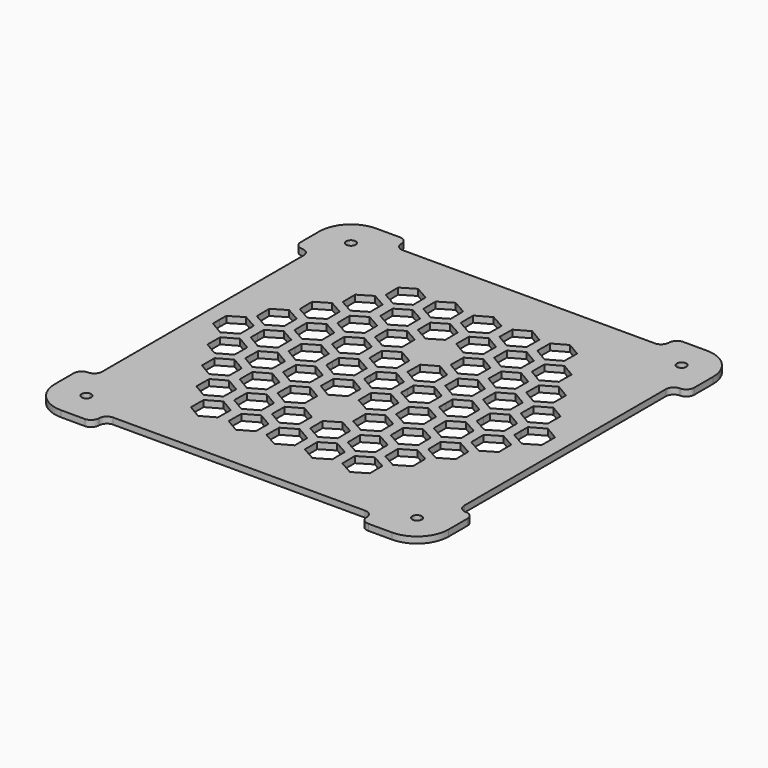
from build123d import *

# Parameters (mm, degrees)
F2_DEPTH = 2
F3_DEPTH = 2
F4_DEPTH = 2
F5_R     = 2.49999
F6_R     = 10


# Not quite as in the source:
# - a fillet or chamfer is up to 0.001 mm smaller than in the source, because OpenCascade refuses the exact size


with BuildPart() as f2:
    # F0 (on Top) → F2 (new body)
    with BuildSketch(Plane.XY):
        Polygon((-57.5, -57.5), (-57.5, -42.5), (-62.5, -42.5), (-62.5, -62.5), (-42.5, -62.5), (-42.5, -57.5), align=None)
        with BuildLine():
            Line((-52.5, -51), (-52.5, -42.5))
            Line((-52.5, -42.5), (-57.5, -42.5))
            Line((-57.5, -42.5), (-57.5, -57.5))
            Line((-57.5, -57.5), (-42.5, -57.5))
            Line((-42.5, -57.5), (-42.5, -52.5))
            Line((-42.5, -52.5), (-51, -52.5))
            ThreePointArc((-51, -52.5), (-53.5606601718, -53.5606601718), (-52.5, -51))
        make_face()
        with BuildLine():
            Line((-42.5, -42.5), (-52.5, -42.5))
            Line((-52.5, -42.5), (-52.5, -51))
            ThreePointArc((-52.5, -51), (-51.4393398282, -51.4393398282), (-51, -52.5))
            Line((-51, -52.5), (-42.5, -52.5))
            Line((-42.5, -52.5), (-42.5, -42.5))
        make_face()
        with BuildLine():
            ThreePointArc((1.078e-07, -52.5), (-37.1231059749, -37.1231060497), (-52.5, 2.1e-09))
            Line((-52.5, 2.1e-09), (-52.5, -42.5))
            Line((-52.5, -42.5), (-42.5, -42.5))
            Line((-42.5, -42.5), (-42.5, -52.5))
            Line((-42.5, -52.5), (1.078e-07, -52.5))
        make_face()
        Polygon((42.5, -52.5), (1.078e-07, -52.5), (-42.5, -52.5), (-42.5, -57.5), (42.5, -57.5), align=None)
        with BuildLine():
            Line((57.5, -42.5), (52.5, -42.5))
            Line((52.5, -42.5), (52.5, -51))
            ThreePointArc((52.5, -51), (53.5606601718, -51.4393398282), (54, -52.5))
            ThreePointArc((54, -52.5), (52.5, -54), (51, -52.5))
            Line((51, -52.5), (42.5, -52.5))
            Line((42.5, -52.5), (42.5, -57.5))
            Line((42.5, -57.5), (57.5, -57.5))
            Line((57.5, -57.5), (57.5, -42.5))
        make_face()
        Polygon((62.5, -42.5), (57.5, -42.5), (57.5, -57.5), (42.5, -57.5), (42.5, -62.5), (62.5, -62.5), align=None)
        with BuildLine():
            Line((52.5, -51), (52.5, -42.5))
            Line((52.5, -42.5), (42.5, -42.5))
            Line((42.5, -42.5), (42.5, -52.5))
            Line((42.5, -52.5), (51, -52.5))
            ThreePointArc((51, -52.5), (51.4393398282, -51.4393398282), (52.5, -51))
        make_face()
        Polygon((52.5, 42.5), (52.5, 0), (52.5, -42.5), (57.5, -42.5), (57.5, 42.5), align=None)
        Polygon((42.5, 62.5), (42.5, 57.5), (57.5, 57.5), (57.5, 42.5), (62.5, 42.5), (62.5, 62.5), align=None)
        with BuildLine():
            Line((42.5, 57.5), (42.5, 52.5))
            Line((42.5, 52.5), (51, 52.5))
            ThreePointArc((51, 52.5), (52.5, 54), (54, 52.5))
            ThreePointArc((54, 52.5), (53.5606601718, 51.4393398282), (52.5, 51))
            Line((52.5, 51), (52.5, 42.5))
            Line((52.5, 42.5), (57.5, 42.5))
            Line((57.5, 42.5), (57.5, 57.5))
            Line((57.5, 57.5), (42.5, 57.5))
        make_face()
        with BuildLine():
            Line((51, 52.5), (42.5, 52.5))
            Line((42.5, 52.5), (42.5, 42.5))
            Line((42.5, 42.5), (52.5, 42.5))
            Line((52.5, 42.5), (52.5, 51))
            ThreePointArc((52.5, 51), (51.4393398282, 51.4393398282), (51, 52.5))
        make_face()
        with BuildLine():
            Line((42.5, 52.5), (0, 52.5))
            ThreePointArc((0, 52.5), (37.1231060123, 37.1231060123), (52.5, 0))
            Line((52.5, 0), (52.5, 42.5))
            Line((52.5, 42.5), (42.5, 42.5))
            Line((42.5, 42.5), (42.5, 52.5))
        make_face()
        with BuildLine():
            ThreePointArc((-52.5, 51), (-53.5606601718, 53.5606601718), (-51, 52.5))
            Line((-51, 52.5), (-42.5, 52.5))
            Line((-42.5, 52.5), (-42.5, 57.5))
            Line((-42.5, 57.5), (-57.5, 57.5))
            Line((-57.5, 57.5), (-57.5, 42.5))
            Line((-57.5, 42.5), (-52.5, 42.5))
            Line((-52.5, 42.5), (-52.5, 51))
        make_face()
        Polygon((-52.5, 2.1e-09), (-52.5, 42.5), (-57.5, 42.5), (-57.5, -42.5), (-52.5, -42.5), align=None)
        with BuildLine():
            Line((0, 52.5), (-42.5, 52.5))
            Line((-42.5, 52.5), (-42.5, 42.5))
            Line((-42.5, 42.5), (-52.5, 42.5))
            Line((-52.5, 42.5), (-52.5, 2.1e-09))
            ThreePointArc((-52.5, 2.1e-09), (-37.1231060115, 37.123106013), (0, 52.5))
        make_face()
        Polygon((-42.5, 57.5), (-42.5, 52.5), (0, 52.5), (42.5, 52.5), (42.5, 57.5), align=None)
        with BuildLine():
            Line((-42.5, 52.5), (-51, 52.5))
            ThreePointArc((-51, 52.5), (-51.4393398282, 51.4393398282), (-52.5, 51))
            Line((-52.5, 51), (-52.5, 42.5))
            Line((-52.5, 42.5), (-42.5, 42.5))
            Line((-42.5, 42.5), (-42.5, 52.5))
        make_face()
        with BuildLine():
            Line((52.5, -42.5), (52.5, 0))
            ThreePointArc((52.5, 0), (37.1231060504, -37.1231059742), (1.078e-07, -52.5))
            Line((1.078e-07, -52.5), (42.5, -52.5))
            Line((42.5, -52.5), (42.5, -42.5))
            Line((42.5, -42.5), (52.5, -42.5))
        make_face()
        with BuildLine():
            ThreePointArc((52.5, 0), (37.1231060123, 37.1231060123), (0, 52.5))
            ThreePointArc((0, 52.5), (-37.1231060115, 37.123106013), (-52.5, 2.1e-09))
            ThreePointArc((-52.5, 2.1e-09), (-37.1231059749, -37.1231060497), (1.078e-07, -52.5))
            ThreePointArc((1.078e-07, -52.5), (37.1231060504, -37.1231059742), (52.5, 0))
        make_face()
    extrude(amount=F2_DEPTH)

    # F0 (on Top) + F1 (on face) → F3 (join)
    with BuildSketch(Plane.XY):
        Polygon((-57.5, 57.5), (-42.5, 57.5), (-42.5, 62.5), (-62.5, 62.5), (-62.5, 42.5), (-57.5, 42.5), align=None)
        Polygon((-42.5, 57.5), (-42.5, 52.5), (0, 52.5), (42.5, 52.5), (42.5, 57.5), align=None)
        with BuildLine():
            ThreePointArc((-52.5, 51), (-53.5606601718, 53.5606601718), (-51, 52.5))
            Line((-51, 52.5), (-42.5, 52.5))
            Line((-42.5, 52.5), (-42.5, 57.5))
            Line((-42.5, 57.5), (-57.5, 57.5))
            Line((-57.5, 57.5), (-57.5, 42.5))
            Line((-57.5, 42.5), (-52.5, 42.5))
            Line((-52.5, 42.5), (-52.5, 51))
        make_face()
        with BuildLine():
            Line((-42.5, 52.5), (-51, 52.5))
            ThreePointArc((-51, 52.5), (-51.4393398282, 51.4393398282), (-52.5, 51))
            Line((-52.5, 51), (-52.5, 42.5))
            Line((-52.5, 42.5), (-42.5, 42.5))
            Line((-42.5, 42.5), (-42.5, 52.5))
        make_face()
        with BuildLine():
            Line((0, 52.5), (-42.5, 52.5))
            Line((-42.5, 52.5), (-42.5, 42.5))
            Line((-42.5, 42.5), (-52.5, 42.5))
            Line((-52.5, 42.5), (-52.5, 2.1e-09))
            ThreePointArc((-52.5, 2.1e-09), (-37.1231060115, 37.123106013), (0, 52.5))
        make_face()
        with BuildLine():
            Line((51, 52.5), (42.5, 52.5))
            Line((42.5, 52.5), (42.5, 42.5))
            Line((42.5, 42.5), (52.5, 42.5))
            Line((52.5, 42.5), (52.5, 51))
            ThreePointArc((52.5, 51), (51.4393398282, 51.4393398282), (51, 52.5))
        make_face()
        with BuildLine():
            Line((42.5, 57.5), (42.5, 52.5))
            Line((42.5, 52.5), (51, 52.5))
            ThreePointArc((51, 52.5), (52.5, 54), (54, 52.5))
            ThreePointArc((54, 52.5), (53.5606601718, 51.4393398282), (52.5, 51))
            Line((52.5, 51), (52.5, 42.5))
            Line((52.5, 42.5), (57.5, 42.5))
            Line((57.5, 42.5), (57.5, 57.5))
            Line((57.5, 57.5), (42.5, 57.5))
        make_face()
        Polygon((42.5, 62.5), (42.5, 57.5), (57.5, 57.5), (57.5, 42.5), (62.5, 42.5), (62.5, 62.5), align=None)
        with BuildLine():
            Line((42.5, 52.5), (0, 52.5))
            ThreePointArc((0, 52.5), (37.1231060123, 37.1231060123), (52.5, 0))
            Line((52.5, 0), (52.5, 42.5))
            Line((52.5, 42.5), (42.5, 42.5))
            Line((42.5, 42.5), (42.5, 52.5))
        make_face()
        Polygon((52.5, 42.5), (52.5, 0), (52.5, -42.5), (57.5, -42.5), (57.5, 42.5), align=None)
        with BuildLine():
            Line((52.5, -51), (52.5, -42.5))
            Line((52.5, -42.5), (42.5, -42.5))
            Line((42.5, -42.5), (42.5, -52.5))
            Line((42.5, -52.5), (51, -52.5))
            ThreePointArc((51, -52.5), (51.4393398282, -51.4393398282), (52.5, -51))
        make_face()
        with BuildLine():
            Line((57.5, -42.5), (52.5, -42.5))
            Line((52.5, -42.5), (52.5, -51))
            ThreePointArc((52.5, -51), (53.5606601718, -51.4393398282), (54, -52.5))
            ThreePointArc((54, -52.5), (52.5, -54), (51, -52.5))
            Line((51, -52.5), (42.5, -52.5))
            Line((42.5, -52.5), (42.5, -57.5))
            Line((42.5, -57.5), (57.5, -57.5))
            Line((57.5, -57.5), (57.5, -42.5))
        make_face()
        Polygon((62.5, -42.5), (57.5, -42.5), (57.5, -57.5), (42.5, -57.5), (42.5, -62.5), (62.5, -62.5), align=None)
        Polygon((42.5, -52.5), (1.078e-07, -52.5), (-42.5, -52.5), (-42.5, -57.5), (42.5, -57.5), align=None)
        with BuildLine():
            ThreePointArc((1.078e-07, -52.5), (-37.1231059749, -37.1231060497), (-52.5, 2.1e-09))
            Line((-52.5, 2.1e-09), (-52.5, -42.5))
            Line((-52.5, -42.5), (-42.5, -42.5))
            Line((-42.5, -42.5), (-42.5, -52.5))
            Line((-42.5, -52.5), (1.078e-07, -52.5))
        make_face()
        Polygon((-52.5, 2.1e-09), (-52.5, 42.5), (-57.5, 42.5), (-57.5, -42.5), (-52.5, -42.5), align=None)
        with BuildLine():
            Line((-52.5, -51), (-52.5, -42.5))
            Line((-52.5, -42.5), (-57.5, -42.5))
            Line((-57.5, -42.5), (-57.5, -57.5))
            Line((-57.5, -57.5), (-42.5, -57.5))
            Line((-42.5, -57.5), (-42.5, -52.5))
            Line((-42.5, -52.5), (-51, -52.5))
            ThreePointArc((-51, -52.5), (-53.5606601718, -53.5606601718), (-52.5, -51))
        make_face()
        Polygon((-57.5, -57.5), (-57.5, -42.5), (-62.5, -42.5), (-62.5, -62.5), (-42.5, -62.5), (-42.5, -57.5), align=None)
        with BuildLine():
            Line((-42.5, -42.5), (-52.5, -42.5))
            Line((-52.5, -42.5), (-52.5, -51))
            ThreePointArc((-52.5, -51), (-51.4393398282, -51.4393398282), (-51, -52.5))
            Line((-51, -52.5), (-42.5, -52.5))
            Line((-42.5, -52.5), (-42.5, -42.5))
        make_face()
        with BuildLine():
            Line((52.5, -42.5), (52.5, 0))
            ThreePointArc((52.5, 0), (37.1231060504, -37.1231059742), (1.078e-07, -52.5))
            Line((1.078e-07, -52.5), (42.5, -52.5))
            Line((42.5, -52.5), (42.5, -42.5))
            Line((42.5, -42.5), (52.5, -42.5))
        make_face()
    with BuildSketch(Plane.XY):
        with BuildLine():
            ThreePointArc((1.078e-07, -52.5), (37.1231060504, -37.1231059742), (52.5, 0))
            ThreePointArc((52.5, 0), (37.1231060123, 37.1231060123), (0, 52.5))
            ThreePointArc((0, 52.5), (-37.1231060115, 37.123106013), (-52.5, 2.1e-09))
            ThreePointArc((-52.5, 2.1e-09), (-37.1231059749, -37.1231060497), (1.078e-07, -52.5))
        make_face()
        Polygon((-30.0605619615, -34.0471505219), (-34.3618349463, -31.497826943), (-34.3046924569, -26.4981534801), (-29.9462769826, -24.0478035961), (-25.6450039978, -26.597127175), (-25.7021464872, -31.5968006379), align=None, mode=Mode.SUBTRACT)
        Polygon((-19.7023299459, -36.2189863238), (-19.7594724353, -41.2186597867), (-24.1178879095, -43.6690096707), (-28.4191608943, -41.1196860918), (-28.3620184049, -36.1200126289), (-24.0036029307, -33.6696627449), align=None, mode=Mode.SUBTRACT)
        Polygon((-13.6871435908, -26.5516522719), (-13.7442860802, -31.5513257348), (-18.1027015545, -34.0016756188), (-22.4039745393, -31.4523520399), (-22.3468320499, -26.4526785769), (-17.9884165756, -24.0023286929), align=None, mode=Mode.SUBTRACT)
        Polygon((-12.1600275025, -43.6235347676), (-16.4613004873, -41.0742111886), (-16.4041579979, -36.0745377257), (-12.0457425237, -33.6241878417), (-7.7444695389, -36.1735114207), (-7.8016120283, -41.1731848836), align=None, mode=Mode.SUBTRACT)
        Polygon((-6.0305561687, -23.9568537898), (-1.7292831839, -26.5061773687), (-1.7864256733, -31.5058508316), (-6.1448411475, -33.9562007156), (-10.4461141323, -31.4068771367), (-10.3889716429, -26.4072036738), align=None, mode=Mode.SUBTRACT)
        Polygon((-36.0032360134, -24.4252913731), (-40.3045089982, -21.8759677942), (-40.2473665088, -16.8762943313), (-35.8889510346, -14.4259444473), (-31.5876780498, -16.9752680262), (-31.6448205392, -21.9749414892), align=None, mode=Mode.SUBTRACT)
        Polygon((-41.9459100654, -14.8034322244), (-46.2471830502, -12.2541086454), (-46.1900405608, -7.2544351825), (-41.8316250866, -4.8040852985), (-37.5303521017, -7.3534088774), (-37.5874945912, -12.3530823404), align=None, mode=Mode.SUBTRACT)
        Polygon((-29.9880496584, -14.7579573212), (-34.2893226432, -12.2086337423), (-34.2321801538, -7.2089602793), (-29.8737646796, -4.7586103953), (-25.5724916948, -7.3079339743), (-25.6296341842, -12.3076074372), align=None, mode=Mode.SUBTRACT)
        Polygon((-28.3466485913, -21.8304928911), (-28.2895061018, -16.8308194281), (-23.9310906276, -14.3804695441), (-19.6298176428, -16.9297931231), (-19.6869601322, -21.929466586), (-24.0453756064, -24.37981647), align=None, mode=Mode.SUBTRACT)
        Polygon((-11.9732302206, -14.334994641), (-7.6719572358, -16.8843182199), (-7.7290997252, -21.8839916828), (-12.0875151995, -24.3343415668), (-16.3887881843, -21.7850179879), (-16.3316456949, -16.785344525), align=None, mode=Mode.SUBTRACT)
        Polygon((-22.2743197468, -7.1634853762), (-17.9159042726, -4.7131354922), (-13.6146312878, -7.2624590711), (-13.6717737772, -12.262132534), (-18.0301892514, -14.712482418), (-22.3314622362, -12.1631588391), align=None, mode=Mode.SUBTRACT)
        Polygon((-1.7139133702, -12.2166576309), (-6.0723288444, -14.6670075149), (-10.3736018292, -12.1176839359), (-10.3164593398, -7.118010473), (-5.9580438656, -4.667660589), (-1.6567708808, -7.216984168), align=None, mode=Mode.SUBTRACT)
        Polygon((-4.4462975909, -36.0290628226), (0, -33.4775075316), (4.4462975909, -36.0290628226), (4.5034400803, -41.0287362855), (0, -43.5275360942), (-4.5034400803, -41.0287362855), align=None, mode=Mode.SUBTRACT)
        Polygon((12.1600275025, -43.6235347676), (7.8016120283, -41.1731848836), (7.7444695389, -36.1735114207), (12.0457425237, -33.6241878417), (16.4041579979, -36.0745377257), (16.4613004873, -41.0742111886), align=None, mode=Mode.SUBTRACT)
        Polygon((1.7864256733, -31.5058508316), (1.7292831839, -26.5061773687), (6.0305561687, -23.9568537898), (10.3889716429, -26.4072036738), (10.4461141323, -31.4068771367), (6.1448411475, -33.9562007156), align=None, mode=Mode.SUBTRACT)
        Polygon((24.1178879095, -43.6690096707), (19.7594724353, -41.2186597867), (19.7023299459, -36.2189863238), (24.0036029307, -33.6696627449), (28.3620184049, -36.1200126289), (28.4191608943, -41.1196860918), align=None, mode=Mode.SUBTRACT)
        Polygon((13.7442860802, -31.5513257348), (13.6871435908, -26.5516522719), (17.9884165756, -24.0023286929), (22.3468320499, -26.4526785769), (22.4039745393, -31.4523520399), (18.1027015545, -34.0016756188), align=None, mode=Mode.SUBTRACT)
        Polygon((34.3046924569, -26.4981534801), (34.3618349463, -31.497826943), (30.0605619615, -34.0471505219), (25.7021464872, -31.5968006379), (25.6450039978, -26.597127175), (29.9462769826, -24.0478035961), align=None, mode=Mode.SUBTRACT)
        Polygon((7.6719572358, -16.8843182199), (11.9732302206, -14.334994641), (16.3316456949, -16.785344525), (16.3887881843, -21.7850179879), (12.0875151995, -24.3343415668), (7.7290997252, -21.8839916828), align=None, mode=Mode.SUBTRACT)
        Polygon((28.2895061018, -16.8308194281), (28.3466485913, -21.8304928911), (24.0453756064, -24.37981647), (19.6869601322, -21.929466586), (19.6298176428, -16.9297931231), (23.9310906276, -14.3804695441), align=None, mode=Mode.SUBTRACT)
        Polygon((5.9580438656, -4.667660589), (10.3164593398, -7.118010473), (10.3736018292, -12.1176839359), (6.0723288444, -14.6670075149), (1.7139133702, -12.2166576309), (1.6567708808, -7.216984168), align=None, mode=Mode.SUBTRACT)
        Polygon((22.2743197468, -7.1634853762), (22.3314622362, -12.1631588391), (18.0301892514, -14.712482418), (13.6717737772, -12.262132534), (13.6146312878, -7.2624590711), (17.9159042726, -4.7131354922), align=None, mode=Mode.SUBTRACT)
        Polygon((36.0032360134, -24.4252913731), (31.6448205392, -21.9749414892), (31.5876780498, -16.9752680262), (35.8889510346, -14.4259444473), (40.2473665088, -16.8762943313), (40.3045089982, -21.8759677942), align=None, mode=Mode.SUBTRACT)
        Polygon((34.2893226432, -12.2086337423), (29.9880496584, -14.7579573212), (25.6296341842, -12.3076074372), (25.5724916948, -7.3079339743), (29.8737646796, -4.7586103953), (34.2321801538, -7.2089602793), align=None, mode=Mode.SUBTRACT)
        Polygon((46.1900405608, -7.2544351825), (46.2471830502, -12.2541086454), (41.9459100654, -14.8034322244), (37.5874945912, -12.3530823404), (37.5303521017, -7.3534088774), (41.8316250866, -4.8040852985), align=None, mode=Mode.SUBTRACT)
        Polygon((-52.2273667157, 0), (-52.1898571022, 2.6322494966), (-47.8885841173, 5.1815730756), (-43.5301686431, 2.7312231916), (-43.5139536858, 0), (-43.5301686431, -2.7312231916), (-47.8885841173, -5.1815730756), (-52.1898571022, -2.6322494966), align=None, mode=Mode.SUBTRACT)
        Polygon((-46.1900405608, 7.2544351825), (-46.2471830502, 12.2541086454), (-41.9459100654, 14.8034322244), (-37.5874945912, 12.3530823404), (-37.5303521017, 7.3534088774), (-41.8316250866, 4.8040852985), align=None, mode=Mode.SUBTRACT)
        Polygon((-40.2213297784, 0), (-40.2319966952, 2.5867745935), (-35.9307237104, 5.1360981724), (-31.5723082361, 2.6857482884), (-31.5532833338, 0), (-31.5723082361, -2.6857482884), (-35.9307237104, -5.1360981724), (-40.2319966952, -2.5867745935), align=None, mode=Mode.SUBTRACT)
        Polygon((-34.2321801538, 7.2089602793), (-34.2893226432, 12.2086337423), (-29.9880496584, 14.7579573212), (-25.6296341842, 12.3076074372), (-25.5724916948, 7.3079339743), (-29.8737646796, 4.7586103953), align=None, mode=Mode.SUBTRACT)
        Polygon((-40.2473665088, 16.8762943313), (-40.3045089982, 21.8759677942), (-36.0032360134, 24.4252913731), (-31.6448205392, 21.9749414892), (-31.5876780498, 16.9752680262), (-35.8889510346, 14.4259444473), align=None, mode=Mode.SUBTRACT)
        Polygon((-28.2807368785, 0), (-28.2741362882, 2.5412996903), (-23.9728633034, 5.0906232692), (-19.6144478292, 2.6402733852), (-19.6275580674, 0), (-19.6144478292, -2.6402733852), (-23.9728633034, -5.0906232692), (-28.2741362882, -2.5412996903), align=None, mode=Mode.SUBTRACT)
        Polygon((-22.2743197468, 7.1634853762), (-22.3314622362, 12.1631588391), (-18.0301892514, 14.712482418), (-13.6717737772, 12.262132534), (-13.6146312878, 7.2624590711), (-17.9159042726, 4.7131354922), align=None, mode=Mode.SUBTRACT)
        Polygon((-16.3349322975, 0), (-16.3162758812, 2.4958247872), (-12.0150028964, 5.0451483661), (-7.4003737783, 2.4507523084), (-7.4243661948, 0), (-7.4003737783, -2.4507523084), (-12.0150028964, -5.0451483661), (-16.3162758812, -2.4958247872), align=None, mode=Mode.SUBTRACT)
        Polygon((-10.3164593398, 7.118010473), (-10.3736018292, 12.1176839359), (-6.0723288444, 14.6670075149), (-1.7139133702, 12.2166576309), (-1.6567708808, 7.216984168), (-5.9580438656, 4.667660589), align=None, mode=Mode.SUBTRACT)
        Polygon((-28.2895061018, 16.8308194281), (-28.3466485913, 21.8304928911), (-24.0453756064, 24.37981647), (-19.6869601322, 21.929466586), (-19.6298176428, 16.9297931231), (-23.9310906276, 14.3804695441), align=None, mode=Mode.SUBTRACT)
        Polygon((-16.3316456949, 16.785344525), (-16.3887881843, 21.7850179879), (-12.0875151995, 24.3343415668), (-7.7290997252, 21.8839916828), (-7.6719572358, 16.8843182199), (-11.9732302206, 14.334994641), align=None, mode=Mode.SUBTRACT)
        Polygon((-34.3046924569, 26.4981534801), (-34.3618349463, 31.497826943), (-30.0605619615, 34.0471505219), (-25.7021464872, 31.5968006379), (-25.6450039978, 26.597127175), (-29.9462769826, 24.0478035961), align=None, mode=Mode.SUBTRACT)
        Polygon((-22.3468320499, 26.4526785769), (-22.4039745393, 31.4523520399), (-18.1027015545, 34.0016756188), (-13.7442860802, 31.5513257348), (-13.6871435908, 26.5516522719), (-17.9884165756, 24.0023286929), align=None, mode=Mode.SUBTRACT)
        Polygon((-28.3620184049, 36.1200126289), (-28.4191608943, 41.1196860918), (-24.1178879095, 43.6690096707), (-19.7594724353, 41.2186597867), (-19.7023299459, 36.2189863238), (-24.0036029307, 33.6696627449), align=None, mode=Mode.SUBTRACT)
        Polygon((-10.3889716429, 26.4072036738), (-10.4461141323, 31.4068771367), (-6.1448411475, 33.9562007156), (-1.7864256733, 31.5058508316), (-1.7292831839, 26.5061773687), (-6.0305561687, 23.9568537898), align=None, mode=Mode.SUBTRACT)
        Polygon((-16.4041579979, 36.0745377257), (-16.4613004873, 41.0742111886), (-12.1600275025, 43.6235347676), (-7.8016120283, 41.1731848836), (-7.7444695389, 36.1735114207), (-12.0457425237, 33.6241878417), align=None, mode=Mode.SUBTRACT)
        Polygon((-4.3574729934, 0), (-4.3584154742, 2.450349884), (0, 5.0096325576), (4.3584154742, 2.450349884), (4.3574729934, 0), (4.3584154742, -2.450349884), (0, -5.0096325576), (-4.3584154742, -2.450349884), align=None, mode=Mode.SUBTRACT)
        Polygon((7.4243661948, 0), (7.4003737783, 2.4507523084), (12.0150028964, 5.0451483661), (16.3162758812, 2.4958247872), (16.3349322975, 0), (16.3162758812, -2.4958247872), (12.0150028964, -5.0451483661), (7.4003737783, -2.4507523084), align=None, mode=Mode.SUBTRACT)
        Polygon((6.0723288444, 14.6670075149), (10.3736018292, 12.1176839359), (10.3164593398, 7.118010473), (5.9580438656, 4.667660589), (1.6567708808, 7.216984168), (1.7139133702, 12.2166576309), align=None, mode=Mode.SUBTRACT)
        Polygon((19.6275580674, 0), (19.6144478292, 2.6402733852), (23.9728633034, 5.0906232692), (28.2741362882, 2.5412996903), (28.2807368785, 0), (28.2741362882, -2.5412996903), (23.9728633034, -5.0906232692), (19.6144478292, -2.6402733852), align=None, mode=Mode.SUBTRACT)
        Polygon((22.2743197468, 7.1634853762), (17.9159042726, 4.7131354922), (13.6146312878, 7.2624590711), (13.6717737772, 12.262132534), (18.0301892514, 14.712482418), (22.3314622362, 12.1631588391), align=None, mode=Mode.SUBTRACT)
        Polygon((12.0875151995, 24.3343415668), (16.3887881843, 21.7850179879), (16.3316456949, 16.785344525), (11.9732302206, 14.334994641), (7.6719572358, 16.8843182199), (7.7290997252, 21.8839916828), align=None, mode=Mode.SUBTRACT)
        Polygon((24.0453756064, 24.37981647), (28.3466485913, 21.8304928911), (28.2895061018, 16.8308194281), (23.9310906276, 14.3804695441), (19.6298176428, 16.9297931231), (19.6869601322, 21.929466586), align=None, mode=Mode.SUBTRACT)
        Polygon((40.2319966952, 2.5867745935), (40.2213297784, 0), (40.2319966952, -2.5867745935), (35.9307237104, -5.1360981724), (31.5723082361, -2.6857482884), (31.5532833338, 0), (31.5723082361, 2.6857482884), (35.9307237104, 5.1360981724), align=None, mode=Mode.SUBTRACT)
        Polygon((29.8737646796, 4.7586103953), (25.5724916948, 7.3079339743), (25.6296341842, 12.3076074372), (29.9880496584, 14.7579573212), (34.2893226432, 12.2086337423), (34.2321801538, 7.2089602793), align=None, mode=Mode.SUBTRACT)
        Polygon((43.5139536858, 0), (43.5301686431, 2.7312231916), (47.8885841173, 5.1815730756), (52.1898571022, 2.6322494966), (52.2273667157, 0), (52.1898571022, -2.6322494966), (47.8885841173, -5.1815730756), (43.5301686431, -2.7312231916), align=None, mode=Mode.SUBTRACT)
        Polygon((46.1900405608, 7.2544351825), (41.8316250866, 4.8040852985), (37.5303521017, 7.3534088774), (37.5874945912, 12.3530823404), (41.9459100654, 14.8034322244), (46.2471830502, 12.2541086454), align=None, mode=Mode.SUBTRACT)
        Polygon((40.3045089982, 21.8759677942), (40.2473665088, 16.8762943313), (35.8889510346, 14.4259444473), (31.5876780498, 16.9752680262), (31.6448205392, 21.9749414892), (36.0032360134, 24.4252913731), align=None, mode=Mode.SUBTRACT)
        Polygon((1.7292831839, 26.5061773687), (1.7864256733, 31.5058508316), (6.1448411475, 33.9562007156), (10.4461141323, 31.4068771367), (10.3889716429, 26.4072036738), (6.0305561687, 23.9568537898), align=None, mode=Mode.SUBTRACT)
        Polygon((-4.4462975909, 36.0290628226), (-4.5034400803, 41.0287362855), (0, 43.5275360942), (4.5034400803, 41.0287362855), (4.4462975909, 36.0290628226), (0, 33.4775075316), align=None, mode=Mode.SUBTRACT)
        Polygon((7.8016120283, 41.1731848836), (12.1600275025, 43.6235347676), (16.4613004873, 41.0742111886), (16.4041579979, 36.0745377257), (12.0457425237, 33.6241878417), (7.7444695389, 36.1735114207), align=None, mode=Mode.SUBTRACT)
        Polygon((22.3468320499, 26.4526785769), (17.9884165756, 24.0023286929), (13.6871435908, 26.5516522719), (13.7442860802, 31.5513257348), (18.1027015545, 34.0016756188), (22.4039745393, 31.4523520399), align=None, mode=Mode.SUBTRACT)
        Polygon((28.3620184049, 36.1200126289), (24.0036029307, 33.6696627449), (19.7023299459, 36.2189863238), (19.7594724353, 41.2186597867), (24.1178879095, 43.6690096707), (28.4191608943, 41.1196860918), align=None, mode=Mode.SUBTRACT)
        Polygon((25.7021464872, 31.5968006379), (30.0605619615, 34.0471505219), (34.3618349463, 31.497826943), (34.3046924569, 26.4981534801), (29.9462769826, 24.0478035961), (25.6450039978, 26.597127175), align=None, mode=Mode.SUBTRACT)
    extrude(amount=-F3_DEPTH)

    # F4 (cut): a face of the model
    f4_faces = [f2.faces().sort_by_distance(p)[0] for p in [
        (0.710552028, -0.710552028, 2),
    ]]
    extrude(f4_faces, amount=-F4_DEPTH, mode=Mode.SUBTRACT)

    # F5 (radius 2.5 in the source; OpenCascade refuses exactly that, so slightly less here)
    f5_edges = [f2.edges().sort_by_distance(p)[0] for p in [
        (-42.5, 57.5, -1),
        (-42.5, 62.5, -1),
        (42.5, 57.5, -1),
        (42.5, 62.5, -1),
        (62.5, 42.5, -1),
        (57.5, 42.5, -1),
        (42.5, -62.5, -1),
        (42.5, -57.5, -1),
        (-62.5, -42.5, -1),
        (-57.5, -42.5, -1),
        (-57.5, 42.5, -1),
        (-62.5, 42.5, -1),
        (-42.5, -62.5, -1),
        (-42.5, -57.5, -1),
        (57.5, -42.5, -1),
        (62.5, -42.5, -1),
    ]]
    fillet(f5_edges, radius=F5_R)

    # F6
    f6_edges = [f2.edges().sort_by_distance(p)[0] for p in [
        (-62.5, 62.5, -1),
        (62.5, 62.5, -1),
        (62.5, -62.5, -1),
        (-62.5, -62.5, -1),
    ]]
    fillet(f6_edges, radius=F6_R)


solid = f2.part
